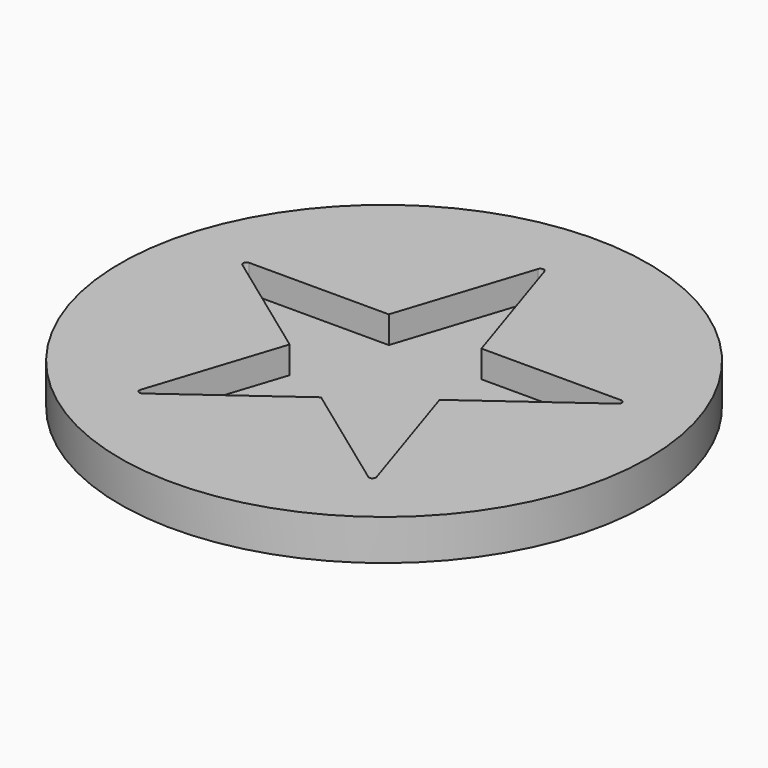
from build123d import *

# Parameters (mm, degrees)
F0_R     = 19.5
F1_DEPTH = 3
F2_DEPTH = 1


# Not quite as in the source:
# - a feature names something its author has since deleted; it is built from what else it names


with BuildPart() as f1:
    # F0 (on Top) → F1 (new body)
    with BuildSketch(Plane.XY):
        with Locations((6.52368e-05, -6.45803e-05)):
            Circle(F0_R)
        with BuildLine():
            ThreePointArc((-8.3389530288, -11.8822470528), (-8.632845655, -11.8822470528), (-8.723663471, -11.6027385556))
            Line((-8.723663471, -11.6027385556), (-5.5384419263, -1.7996346453))
            Line((-5.5384419263, -1.7996346453), (-13.877460192, 4.2590167665))
            ThreePointArc((-13.877460192, 4.2590167665), (-13.968278008, 4.5385252636), (-13.7305138789, 4.7112710151))
            Line((-13.7305138789, 4.7112710151), (-3.4229204369, 4.7112710151))
            Line((-3.4229204369, 4.7112710151), (-0.2376988922, 14.5143749254))
            ThreePointArc((-0.2376988922, 14.5143749254), (6.52368e-05, 14.6871206768), (0.2378293659, 14.5143749254))
            Line((0.2378293659, 14.5143749254), (3.4230509106, 4.7112710151))
            Line((3.4230509106, 4.7112710151), (13.7306443525, 4.7112710151))
            ThreePointArc((13.7306443525, 4.7112710151), (13.9684084816, 4.5385252637), (13.8775906656, 4.2590167665))
            Line((13.8775906656, 4.2590167665), (5.5385724, -1.7996346453))
            Line((5.5385724, -1.7996346453), (8.7237939446, -11.6027385556))
            ThreePointArc((8.7237939446, -11.6027385556), (8.6329761286, -11.8822470528), (8.3390835025, -11.8822470528))
            Line((8.3390835025, -11.8822470528), (6.52368e-05, -5.823595641))
            Line((6.52368e-05, -5.823595641), (-8.3389530288, -11.8822470528))
        make_face(mode=Mode.SUBTRACT)
    extrude(amount=F1_DEPTH)

    # F0 (on Top) → F2 (join)
    with BuildSketch(Plane.XY):
        with BuildLine():
            Line((-5.5384419263, -1.7996346453), (-8.723663471, -11.6027385556))
            ThreePointArc((-8.723663471, -11.6027385556), (-8.632845655, -11.8822470528), (-8.3389530288, -11.8822470528))
            Line((-8.3389530288, -11.8822470528), (6.52368e-05, -5.823595641))
            Line((6.52368e-05, -5.823595641), (-5.5384419263, -1.7996346453))
        make_face()
        with BuildLine():
            Line((-13.877460192, 4.2590167665), (-5.5384419263, -1.7996346453))
            Line((-5.5384419263, -1.7996346453), (-3.4229204369, 4.7112710151))
            Line((-3.4229204369, 4.7112710151), (-13.7305138789, 4.7112710151))
            ThreePointArc((-13.7305138789, 4.7112710151), (-13.968278008, 4.5385252636), (-13.877460192, 4.2590167665))
        make_face()
        Polygon((-3.4229204369, 4.7112710151), (-5.5384419263, -1.7996346453), (6.52368e-05, -5.823595641), (5.5385724, -1.7996346453), (3.4230509106, 4.7112710151), align=None)
        with BuildLine():
            Line((-0.2376988922, 14.5143749254), (-3.4229204369, 4.7112710151))
            Line((-3.4229204369, 4.7112710151), (3.4230509106, 4.7112710151))
            Line((3.4230509106, 4.7112710151), (0.2378293659, 14.5143749254))
            ThreePointArc((0.2378293659, 14.5143749254), (6.52368e-05, 14.6871206768), (-0.2376988922, 14.5143749254))
        make_face()
        with BuildLine():
            Line((5.5385724, -1.7996346453), (6.52368e-05, -5.823595641))
            Line((6.52368e-05, -5.823595641), (8.3390835025, -11.8822470528))
            ThreePointArc((8.3390835025, -11.8822470528), (8.6329761286, -11.8822470528), (8.7237939446, -11.6027385556))
            Line((8.7237939446, -11.6027385556), (5.5385724, -1.7996346453))
        make_face()
        with BuildLine():
            Line((13.7306443525, 4.7112710151), (3.4230509106, 4.7112710151))
            Line((3.4230509106, 4.7112710151), (5.5385724, -1.7996346453))
            Line((5.5385724, -1.7996346453), (13.8775906656, 4.2590167665))
            ThreePointArc((13.8775906656, 4.2590167665), (13.9684084816, 4.5385252637), (13.7306443525, 4.7112710151))
        make_face()
    extrude(amount=F2_DEPTH)


solid = f1.part
